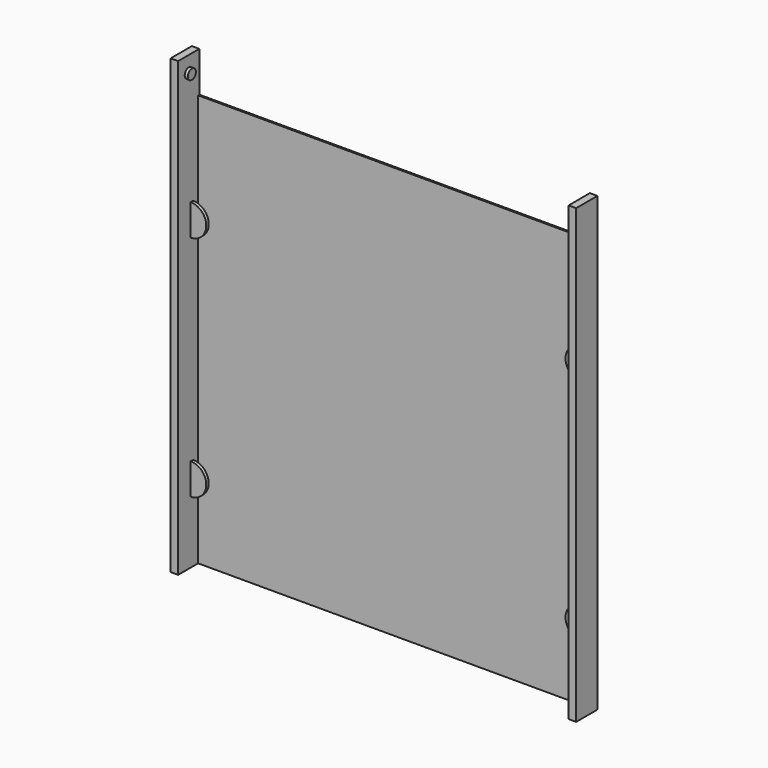
from build123d import *

# Parameters (mm, degrees)
F0_W      = 1.2
F0_H      = 131.87
F0_W_2    = 127.4
F1_DEPTH  = 8.5
F2_W      = 125
F2_H      = 131.87
F3_DEPTH  = 8
F4_W      = 2.4
F4_H      = 8.5
F5_DEPTH  = 12.9
F6_R      = 1.6
F7_DEPTH  = 1
F9_DEPTH  = 3
F10_W     = 125
F10_H     = 2
F11_DEPTH = 130


# Not quite as in the source:
# - a pattern or mirror of a feature is missing from the dataset's text; its kind, count and spacing are read off the source's solid


with BuildPart() as f1:
    # F0 (on Front) → F1 (new body)
    with BuildSketch(Plane.XZ):
        with Locations((-64.3, 0)):
            Rectangle(F0_W, F0_H)
        Rectangle(F0_W_2, F0_H)
        with Locations((64.3, 0)):
            Rectangle(F0_W, F0_H)
    extrude(amount=F1_DEPTH)

    # F2 (on face) → F3 (cut)
    with BuildSketch(Plane.XZ.offset(8.5)):
        Rectangle(F2_W, F2_H)
    extrude(amount=-F3_DEPTH, mode=Mode.SUBTRACT)

    # F4 (on face) → F5 (join)
    with BuildSketch(Plane.XY.offset(65.935)):
        with Locations((-63.7, -4.25)):
            Rectangle(F4_W, F4_H)
        with Locations((63.7, -4.25)):
            Rectangle(F4_W, F4_H)
    extrude(amount=F5_DEPTH)

    # F6 (on face) → F7 (join)
    with BuildSketch(Plane.YZ.offset(-62.5)):
        with Locations((-4.25, 73.735)):
            Circle(F6_R)
    f7 = extrude(amount=F7_DEPTH)

    # F7_copies: F7 across plane
    add(f7.mirror(Plane(origin=(0, 0, 0), x_dir=(0, 0, 1), z_dir=(1, 0, 0))))

    # F8 (on face) → F9 (join)
    with BuildSketch(Plane.XZ.offset(0.5)):
        with BuildLine():
            Line((-62.5, -35.935), (-62.5, -45.935))
            ThreePointArc((-62.5, -45.935), (-57.5, -40.935), (-62.5, -35.935))
        make_face()
        with BuildLine():
            Line((-62.5, 37.065), (-62.5, 27.065))
            ThreePointArc((-62.5, 27.065), (-57.5, 32.065), (-62.5, 37.065))
        make_face()
    f9 = extrude(amount=F9_DEPTH)

    # F9_copies: F9 across plane
    add(f9.mirror(Plane(origin=(0, 0, 0), x_dir=(0, 0, 1), z_dir=(1, 0, 0))))

    # F10 (on face) → F11 (cut)
    with BuildSketch(Plane(origin=(0, 0, -65.935), x_dir=(1, 0, 0), z_dir=(0, 0, -1))):
        with Locations((0, 1.5)):
            Rectangle(F10_W, F10_H)
    extrude(amount=-F11_DEPTH, mode=Mode.SUBTRACT)


solid = f1.part
